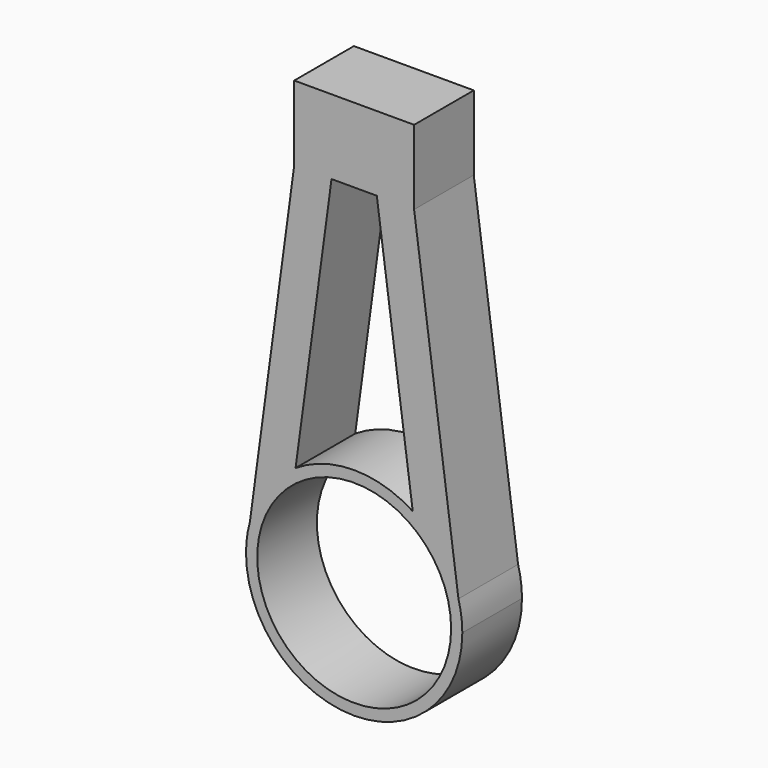
from build123d import *

# Parameters (mm, degrees)
F0_R     = 16.51
F1_DEPTH = 12.7


# Not quite as in the source:
# - a feature names something its author has since deleted; it is built from what else it names


with BuildPart() as f1:
    # F0 (on Front) → F1 (new body)
    with BuildSketch(Plane.XZ):
        with BuildLine():
            ThreePointArc((17.7553829843, 4.8845265973), (14.8425769227, 10.9000062062), (9.9745940638, 15.4796543328))
            ThreePointArc((9.9745940638, 15.4796543328), (0, 18.415), (-9.9745940638, 15.4796543328))
            ThreePointArc((-9.9745940638, 15.4796543328), (-14.8425769227, 10.9000062062), (-17.7553829843, 4.8845265973))
            Line((-17.7553829843, 4.8845265973), (-18.415, 0))
            ThreePointArc((-18.415, 0), (0, -18.415), (18.415, 0))
            Line((18.415, 0), (17.7553829843, 4.8845265973))
        make_face()
        Circle(F0_R, mode=Mode.SUBTRACT)
        with BuildLine():
            ThreePointArc((-17.7553829843, 4.8845265973), (-14.8425769227, 10.9000062062), (-9.9745940638, 15.4796543328))
            Line((-9.9745940638, 15.4796543328), (-3.8560049814, 60.7883871295))
            Line((-3.8560049814, 60.7883871295), (-10.2060049814, 60.7883871295))
            Line((-10.2060049814, 60.7883871295), (-17.7553829843, 4.8845265973))
        make_face()
        with BuildLine():
            Line((3.8560049814, 60.7883871295), (9.9745940638, 15.4796543328))
            ThreePointArc((9.9745940638, 15.4796543328), (14.8425769227, 10.9000062062), (17.7553829843, 4.8845265973))
            Line((17.7553829843, 4.8845265973), (10.2060049814, 60.7883871295))
            Line((10.2060049814, 60.7883871295), (3.8560049814, 60.7883871295))
        make_face()
        with BuildLine():
            ThreePointArc((18.415, 0), (18.2493507098, 2.4644317137), (17.7553829843, 4.8845265973))
            Line((17.7553829843, 4.8845265973), (18.415, 0))
        make_face()
        with BuildLine():
            Line((-18.415, 0), (-17.7553829843, 4.8845265973))
            ThreePointArc((-17.7553829843, 4.8845265973), (-18.2493507098, 2.4644317137), (-18.415, 0))
        make_face()
        Polygon((0, 60.7883871295), (3.8560049814, 60.7883871295), (10.2060049814, 60.7883871295), (10.2060049814, 73.4883871295), (-10.2060049814, 73.4883871295), (-10.2060049814, 60.7883871295), (-3.8560049814, 60.7883871295), align=None)
    extrude(amount=F1_DEPTH)


solid = f1.part
